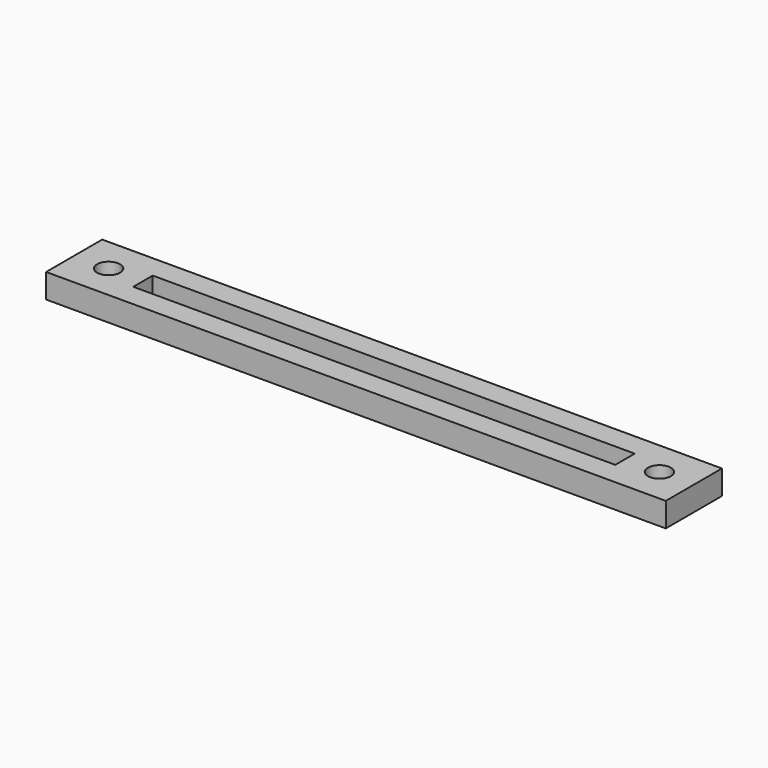
from build123d import *

# Parameters (mm, degrees)
F0_W     = 81
F0_H     = 9.175
F0_R     = 1.5
F1_DEPTH = 3.175


# Not quite as in the source:
# - a length typed as a fraction of an inch, garbled in the dataset ("3 / 203.2 mm" for 3/8 in), is restored


with BuildPart() as f1:
    # F0 (on Top) → F1 (new body)
    with BuildSketch(Plane.XY):
        with Locations((35.4220271409, 16.632870598)):
            Rectangle(F0_W, F0_H)
        with Locations((-0.5779728591, 16.632870598)):
            Circle(F0_R, mode=Mode.SUBTRACT)
        Polygon((3.9220271409, 15.045370598), (3.9220271409, 18.220370598), (35.4220271409, 18.220370598), (66.9220271409, 18.220370598), (66.9220271409, 15.045370598), align=None, mode=Mode.SUBTRACT)
        with Locations((71.4220271409, 16.632870598)):
            Circle(F0_R, mode=Mode.SUBTRACT)
    extrude(amount=F1_DEPTH)


solid = f1.part
